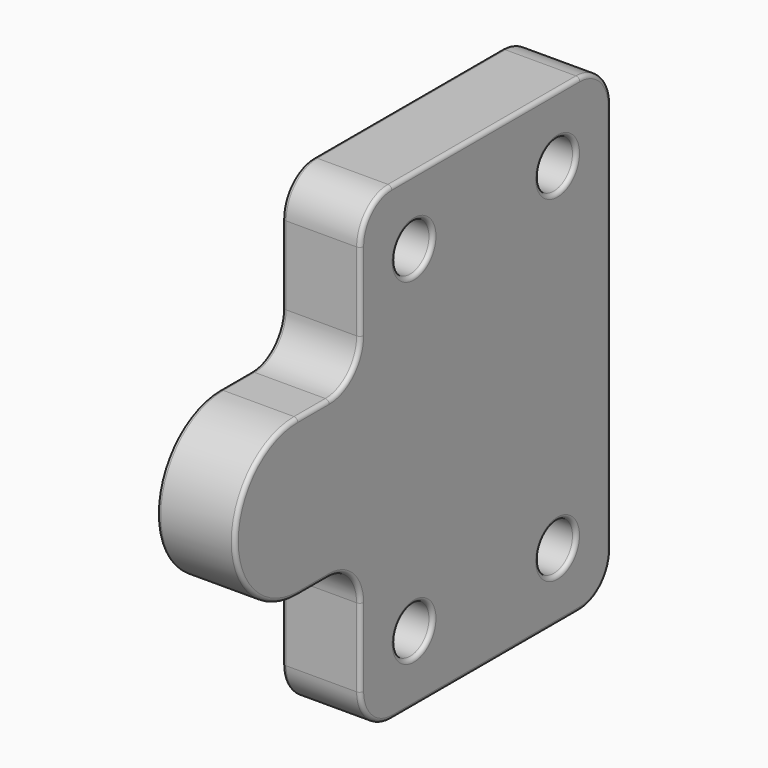
from build123d import *

# Parameters (mm, degrees)
F1_DEPTH = 10
F2_R     = 5
F5_D     = 6
F6_R     = 0.5


with BuildPart() as f1:
    # F0 (on Right) → F1 (new body)
    with BuildSketch(Plane.YZ):
        with BuildLine():
            Line((-20, -15), (-20, -30))
            Line((-20, -30), (20, -30))
            Line((20, -30), (20, 30))
            Line((20, 30), (-20, 30))
            Line((-20, 30), (-20, 15))
            ThreePointArc((-20, 15), (-21.4644660941, 11.4644660941), (-25, 10))
            Line((-25, 10), (-30, 10))
            ThreePointArc((-30, 10), (-40, 0), (-30, -10))
            Line((-30, -10), (-25, -10))
            ThreePointArc((-25, -10), (-21.4644660941, -11.4644660941), (-20, -15))
        make_face()
    extrude(amount=F1_DEPTH)

    # F2
    f2_edges = [f1.edges().sort_by_distance(p)[0] for p in [
        (5, -20, 30),
        (5, 20, 30),
        (5, 20, -30),
        (5, -20, -30),
    ]]
    fillet(f2_edges, radius=F2_R)

    # F5 (through all)
    with Locations(Plane.YZ.offset(10)):
        with Locations((-11.4519952962, 21.4769810358), (11.4519952962, 21.4769810358), (11.4519952962, -21.4769810358), (-11.4519952962, -21.4769810358)):
            Hole(F5_D / 2)

    # F6
    f6_edges = [f1.edges().sort_by_distance(p)[0] for p in [
        (0, -18.535534, -28.535534),
        (5, -20, -25),
        (5, -15, -30),
        (10, -18.535534, -28.535534),
        (0, -18.535534, 28.535534),
        (5, -15, 30),
        (5, -20, 25),
        (10, -18.535534, 28.535534),
        (10, 18.535534, -28.535534),
        (0, 18.535534, 28.535534),
        (5, 20, 25),
        (5, 15, 30),
        (10, 18.535534, 28.535534),
        (5, -30, 10),
        (5, -30, -10),
        (0, -40, 0),
        (10, -40, 0),
        (5, -25, 10),
        (0, -27.5, 10),
        (10, -27.5, 10),
        (0, 0, -30),
        (5, 15, -30),
        (10, 0, -30),
        (0, 0, 30),
        (10, 0, 30),
        (5, -25, -10),
        (0, -27.5, -10),
        (10, -27.5, -10),
        (5, -20, -15),
        (0, -21.464466, -11.464466),
        (10, -21.464466, -11.464466),
        (0, 18.535534, -28.535534),
        (5, 20, -25),
        (0, -20, -20),
        (10, -20, -20),
        (0, 20, 0),
        (10, 20, 0),
        (0, -20, 20),
        (5, -20, 15),
        (10, -20, 20),
        (10, -21.464466, 11.464466),
        (10, -14.451995, -21.476981),
        (10, 8.451995, -21.476981),
        (10, -14.451995, 21.476981),
        (10, 8.451995, 21.476981),
        (0, -21.464466, 11.464466),
        (0, -14.451995, -21.476981),
        (0, 8.451995, -21.476981),
        (0, -14.451995, 21.476981),
        (0, 8.451995, 21.476981),
    ]]
    fillet(f6_edges, radius=F6_R)


solid = f1.part
